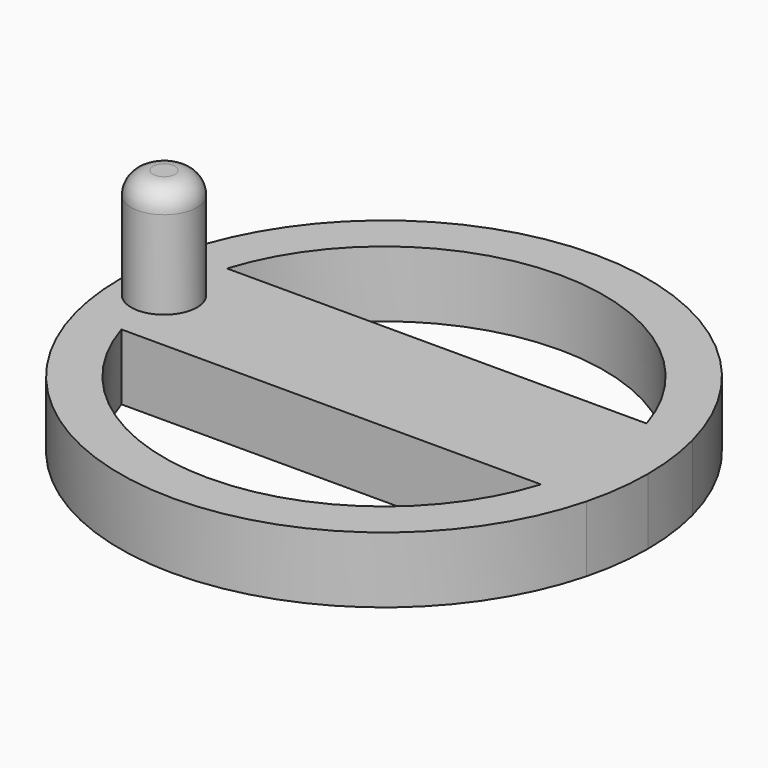
from build123d import *

# Parameters (mm, degrees)
F1_DEPTH = 15
F2_R     = 7.5
F3_DEPTH = 25
F4_R     = 5
F5_W     = 8.242
F5_H     = 12.533
F6_DEPTH = 10


# Not quite as in the source:
# - a feature names something its author has since deleted; it is built from what else it names


with BuildPart() as f1:
    # F0 (on Top) → F1 (new body)
    with BuildSketch(Plane.XY):
        with BuildLine():
            Line((47.6969600708, 15), (58.0947501931, 15))
            ThreePointArc((58.0947501931, 15), (0, 60), (-58.0947501931, 15))
            Line((-58.0947501931, 15), (-47.6969600708, 15))
            ThreePointArc((-47.6969600708, 15), (0, 50), (47.6969600708, 15))
        make_face()
        with BuildLine():
            Line((-47.6969600708, 15), (-58.0947501931, 15))
            ThreePointArc((-58.0947501931, 15), (-60, 0), (-58.0947501931, -15))
            Line((-58.0947501931, -15), (-47.6969600708, -15))
            ThreePointArc((-47.6969600708, -15), (-50, 0), (-47.6969600708, 15))
        make_face()
        with BuildLine():
            ThreePointArc((-58.0947501931, -15), (0, -60), (58.0947501931, -15))
            Line((58.0947501931, -15), (47.6969600708, -15))
            ThreePointArc((47.6969600708, -15), (0, -50), (-47.6969600708, -15))
            Line((-47.6969600708, -15), (-58.0947501931, -15))
        make_face()
        with BuildLine():
            ThreePointArc((58.0947501931, -15), (59.521781776, -7.560257549), (60, 0))
            ThreePointArc((60, 0), (59.521781776, 7.560257549), (58.0947501931, 15))
            Line((58.0947501931, 15), (47.6969600708, 15))
            ThreePointArc((47.6969600708, 15), (49.4208862908, 7.5878849641), (50, 0))
            ThreePointArc((50, 0), (49.4208862908, -7.5878849641), (47.6969600708, -15))
            Line((47.6969600708, -15), (58.0947501931, -15))
        make_face()
        with BuildLine():
            ThreePointArc((50, 0), (49.4208862908, 7.5878849641), (47.6969600708, 15))
            Line((47.6969600708, 15), (-47.6969600708, 15))
            ThreePointArc((-47.6969600708, 15), (-50, 0), (-47.6969600708, -15))
            Line((-47.6969600708, -15), (47.6969600708, -15))
            ThreePointArc((47.6969600708, -15), (49.4208862908, -7.5878849641), (50, 0))
        make_face()
    extrude(amount=F1_DEPTH)

    # F2 (on face) → F3 (join)
    with BuildSketch(Plane.XY.offset(15)):
        with Locations((-50, 0)):
            Circle(F2_R)
    extrude(amount=F3_DEPTH)

    # F4
    f4_edges = [f1.edges().sort_by_distance(p)[0] for p in [
        (-57.5, 0, 40),
    ]]
    fillet(f4_edges, radius=F4_R)

    # F5 (on face) → F6 (cut)
    with BuildSketch(Plane(origin=(0, 0, 0), x_dir=(1, 0, 0), z_dir=(0, 0, -1))):
        Rectangle(F5_W, F5_H)
    extrude(amount=-F6_DEPTH, mode=Mode.SUBTRACT)


solid = f1.part
